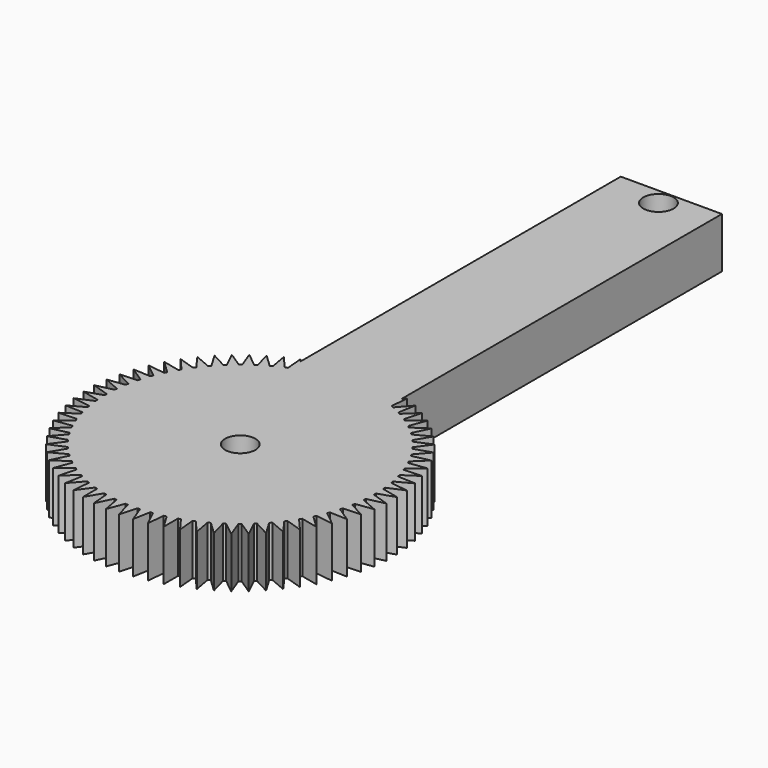
from build123d import *

# Parameters (mm, degrees)
F0_R     = 1.5
F1_DEPTH = 2.5
F3_DEPTH = 5


# Not quite as in the source:
# - a feature names something its author has since deleted; it is built from what else it names
# - the program builds the solid bodies; features that only make, move or delete a surface that nothing else refers to are left out


with BuildPart() as f1:
    # F0 (on Top) → F1 (new body, symmetric)
    with BuildSketch(Plane.XY):
        with BuildLine():
            Line((4.9747981783, 53.2882774979), (-5.0252018217, 53.2882774979))
            Line((-5.0252018217, 53.2882774979), (-5.0252018217, 14.1213197939))
            ThreePointArc((-5.0252018217, 14.1213197939), (-0.0267305738, 14.9880958204), (4.9747981783, 14.1391402048))
            Line((4.9747981783, 14.1391402048), (4.9747981783, 53.2882774979))
        make_face()
        with Locations((0, 51.666546613)):
            Circle(F0_R, mode=Mode.SUBTRACT)
        with BuildLine():
            ThreePointArc((4.9747981783, 14.1391402048), (-0.0267305738, 14.9880958204), (-5.0252018217, 14.1213197939))
            Line((-5.0252018217, 14.1213197939), (-5.0252018217, 13.7012252469))
            Line((-5.0252018217, 13.7012252469), (-5.2664479011, 14.0324002503))
            Line((-5.2664479011, 14.0324002503), (-5.1113713487, 12.2848828663))
            Line((-5.1113713487, 12.2848828663), (-5.35527293, 12.1933450718))
            Line((-5.35527293, 12.1933450718), (-6.5031013908, 13.5038291821))
            Line((-6.5031013908, 13.5038291821), (-6.1920028804, 11.7772477444))
            Line((-6.1920028804, 11.7772477444), (-6.4267172011, 11.6642152849))
            Line((-6.4267172011, 11.6642152849), (-7.6873957319, 12.8665332215))
            Line((-7.6873957319, 12.8665332215), (-7.2227800459, 11.1747891485))
            Line((-7.2227800459, 11.1747891485), (-7.4464173241, 11.0411720949))
            Line((-7.4464173241, 11.0411720949), (-8.8097956827, 12.1256435008))
            Line((-8.8097956827, 12.1256435008), (-8.1954036333, 10.482357721))
            Line((-8.1954036333, 10.482357721), (-8.4061632732, 10.3292318794))
            Line((-8.4061632732, 10.3292318794), (-9.8612643388, 11.2871252283))
            Line((-9.8612643388, 11.2871252283), (-9.1020426494, 9.7055285127))
            Line((-9.1020426494, 9.7055285127), (-9.2982277385, 9.5341267623))
            Line((-9.2982277385, 9.5341267623), (-10.8333358927, 10.3577296603))
            Line((-10.8333358927, 10.3577296603), (-9.9353973701, 8.8505560956))
            Line((-9.9353973701, 8.8505560956), (-10.1154283412, 8.6622584624))
            Line((-10.1154283412, 8.6622584624), (-11.7181837959, 9.3449397433))
            Line((-11.7181837959, 9.3449397433), (-10.6887581131, 7.9243242049))
            Line((-10.6887581131, 7.9243242049), (-10.8511854627, 7.7206467507))
            Line((-10.8511854627, 7.7206467507), (-12.5086837734, 8.2569098662))
            Line((-12.5086837734, 8.2569098662), (-11.3560592606, 6.934290315))
            Line((-11.3560592606, 6.934290315), (-11.4995752192, 6.7168729311))
            Line((-11.4995752192, 6.7168729311), (-13.1984711841, 7.1024002058))
            Line((-13.1984711841, 7.1024002058), (-11.9319280962, 5.8884255969))
            Line((-11.9319280962, 5.8884255969), (-12.0553771577, 5.6590188001))
            Line((-12.0553771577, 5.6590188001), (-13.7819922654, 5.8907061951))
            Line((-13.7819922654, 5.8907061951), (-12.4117280627, 4.7951507382))
            Line((-12.4117280627, 4.7951507382), (-12.5141162878, 4.5556015771))
            Line((-12.5141162878, 4.5556015771), (-14.2545488486, 4.6315836818))
            Line((-14.2545488486, 4.6315836818), (-12.7915960928, 3.6632681452))
            Line((-12.7915960928, 3.6632681452), (-12.8720991118, 3.4155053289))
            Line((-12.8720991118, 3.4155053289), (-14.6123361861, 3.3351703801))
            Line((-14.6123361861, 3.3351703801), (-13.0684737124, 2.5018910711))
            Line((-13.0684737124, 2.5018910711), (-13.1264433623, 2.2479094401))
            Line((-13.1264433623, 2.2479094401), (-14.8524735845, 2.0119042475))
            Line((-14.8524735845, 2.0119042475), (-13.2401316659, 1.3203702412))
            Line((-13.2401316659, 1.3203702412), (-13.2751012091, 1.0622147062))
            Line((-13.2751012091, 1.0622147062), (-14.9730275987, 0.6724394448))
            Line((-14.9730275987, 0.6724394448), (-13.3051878643, 0.1282185665))
            Line((-13.3051878643, 0.1282185665), (-13.3168757467, -0.132032356))
            Line((-13.3168757467, -0.132032356), (-14.9730275987, -0.6724394448))
            Line((-14.9730275987, -0.6724394448), (-13.2631185133, -1.0649654488))
            Line((-13.2631185133, -1.0649654488), (-13.2514306309, -1.3252163712))
            Line((-13.2514306309, -1.3252163712), (-14.8524735845, -2.0119042475))
            Line((-14.8524735845, -2.0119042475), (-13.1142623306, -2.2495749884))
            Line((-13.1142623306, -2.2495749884), (-13.0792927873, -2.5077305234))
            Line((-13.0792927873, -2.5077305234), (-14.6123361861, -3.3351703801))
            Line((-14.6123361861, -3.3351703801), (-12.8598178187, -3.4160722729))
            Line((-12.8598178187, -3.4160722729), (-12.8018481688, -3.670053904))
            Line((-12.8018481688, -3.670053904), (-14.2545488486, -4.6315836818))
            Line((-14.2545488486, -4.6315836818), (-12.5018336152, -4.5550653522))
            Line((-12.5018336152, -4.5550653522), (-12.4213305961, -4.8028281685))
            Line((-12.4213305961, -4.8028281685), (-13.7819922654, -5.8907061951))
            Line((-13.7819922654, -5.8907061951), (-12.0431919983, -5.6573837235))
            Line((-12.0431919983, -5.6573837235), (-11.9408037732, -5.8969328846))
            Line((-11.9408037732, -5.8969328846), (-13.1984711841, -7.1024002058))
            Line((-13.1984711841, -7.1024002058), (-11.4875856808, -6.7141521676))
            Line((-11.4875856808, -6.7141521676), (-11.3641366193, -6.9435589644))
            Line((-11.3641366193, -6.9435589644), (-12.5086837734, -8.2569098662))
            Line((-12.5086837734, -8.2569098662), (-10.839488078, -7.7168622063))
            Line((-10.839488078, -7.7168622063), (-10.6959721194, -7.9342795903))
            Line((-10.6959721194, -7.9342795903), (-11.7181837959, -9.3449397433))
            Line((-11.7181837959, -9.3449397433), (-10.1041172907, -8.657440608))
            Line((-10.1041172907, -8.657440608), (-9.9416899411, -8.8611180621))
            Line((-9.9416899411, -8.8611180621), (-10.8333358927, -10.3577296603))
            Line((-10.8333358927, -10.3577296603), (-9.287394092, -9.5283143883))
            Line((-9.287394092, -9.5283143883), (-9.107363121, -9.7166120216))
            Line((-9.107363121, -9.7166120216), (-9.8612643388, -11.2871252283))
            Line((-9.8612643388, -11.2871252283), (-8.3958942571, -10.3224717838))
            Line((-8.3958942571, -10.3224717838), (-8.1997091681, -10.4938735343))
            Line((-8.1997091681, -10.4938735343), (-8.8097956827, -12.1256435008))
            Line((-8.8097956827, -12.1256435008), (-7.4367956183, -11.033518706))
            Line((-7.4367956183, -11.033518706), (-7.2260359783, -11.1866445476))
            Line((-7.2260359783, -11.1866445476), (-7.6873957319, -12.8665332215))
            Line((-7.6873957319, -12.8665332215), (-6.4178202739, -11.6557302232))
            Line((-6.4178202739, -11.6557302232), (-6.1941829957, -11.7893472767))
            Line((-6.1941829957, -11.7893472767), (-6.5031013908, -13.5038291821))
            Line((-6.5031013908, -13.5038291821), (-5.3471724143, -12.184096654))
            Line((-5.3471724143, -12.184096654), (-5.1124580937, -12.2971291135))
            Line((-5.1124580937, -12.2971291135), (-5.2664479011, -14.0324002503))
            Line((-5.2664479011, -14.0324002503), (-4.2334722666, -12.6143639028))
            Line((-4.2334722666, -12.6143639028), (-3.9895706852, -12.7059016973))
            Line((-3.9895706852, -12.7059016973), (-3.9873920694, -14.4479906826))
            Line((-3.9873920694, -14.4479906826), (-3.0856866893, -12.9430677105))
            Line((-3.0856866893, -12.9430677105), (-2.8345615994, -13.0123738316))
            Line((-2.8345615994, -13.0123738316), (-2.6762321014, -14.7472543892))
            Line((-2.6762321014, -14.7472543892), (-1.9130569772, -13.1675615474))
            Line((-1.9130569772, -13.1675615474), (-1.6567302903, -13.214077983))
            Line((-1.6567302903, -13.214077983), (-1.3435246861, -14.9277818747))
            Line((-1.3435246861, -14.9277818747), (-0.7250244552, -13.2860379212))
            Line((-0.7250244552, -13.2860379212), (-0.465559963, -13.3093901482))
            Line((-0.465559963, -13.3093901482), (0, -14.9881196379))
            Line((0, -14.9881196379), (0.4688455374, -13.2975429296))
            Line((0.4688455374, -13.2975429296), (0.7293587793, -13.2975429296))
            Line((0.7293587793, -13.2975429296), (1.3435246861, -14.9277818747))
            Line((1.3435246861, -14.9277818747), (1.6589406614, -13.2019839413))
            Line((1.6589406614, -13.2019839413), (1.9184051536, -13.1786317143))
            Line((1.9184051536, -13.1786317143), (2.6762321014, -14.7472543892))
            Line((2.6762321014, -14.7472543892), (2.8356789707, -13.0001303408))
            Line((2.8356789707, -13.0001303408), (3.0920056577, -12.9536139053))
            Line((3.0920056577, -12.9536139053), (3.9873920694, -14.4479906826))
            Line((3.9873920694, -14.4479906826), (3.9895860602, -12.6936073349))
            Line((3.9895860602, -12.6936073349), (4.2407111502, -12.6243012138))
            Line((4.2407111502, -12.6243012138), (5.2664479011, -14.0324002503))
            Line((5.2664479011, -14.0324002503), (5.1113713487, -12.2848828663))
            Line((5.1113713487, -12.2848828663), (5.35527293, -12.1933450718))
            Line((5.35527293, -12.1933450718), (6.5031013908, -13.5038291821))
            Line((6.5031013908, -13.5038291821), (6.1920028804, -11.7772477444))
            Line((6.1920028804, -11.7772477444), (6.4267172011, -11.6642152849))
            Line((6.4267172011, -11.6642152849), (7.6873957319, -12.8665332215))
            Line((7.6873957319, -12.8665332215), (7.2227800459, -11.1747891485))
            Line((7.2227800459, -11.1747891485), (7.4464173241, -11.0411720949))
            Line((7.4464173241, -11.0411720949), (8.8097956827, -12.1256435008))
            Line((8.8097956827, -12.1256435008), (8.1954036333, -10.482357721))
            Line((8.1954036333, -10.482357721), (8.4061632732, -10.3292318794))
            Line((8.4061632732, -10.3292318794), (9.8612643388, -11.2871252283))
            Line((9.8612643388, -11.2871252283), (9.1020426494, -9.7055285127))
            Line((9.1020426494, -9.7055285127), (9.2982277385, -9.5341267623))
            Line((9.2982277385, -9.5341267623), (10.8333358927, -10.3577296603))
            Line((10.8333358927, -10.3577296603), (9.9353973701, -8.8505560956))
            Line((9.9353973701, -8.8505560956), (10.1154283412, -8.6622584624))
            Line((10.1154283412, -8.6622584624), (11.7181837959, -9.3449397433))
            Line((11.7181837959, -9.3449397433), (10.6887581131, -7.9243242049))
            Line((10.6887581131, -7.9243242049), (10.8511854627, -7.7206467507))
            Line((10.8511854627, -7.7206467507), (12.5086837734, -8.2569098662))
            Line((12.5086837734, -8.2569098662), (11.3560592606, -6.934290315))
            Line((11.3560592606, -6.934290315), (11.4995752192, -6.7168729311))
            Line((11.4995752192, -6.7168729311), (13.1984711841, -7.1024002058))
            Line((13.1984711841, -7.1024002058), (11.9319280962, -5.8884255969))
            Line((11.9319280962, -5.8884255969), (12.0553771577, -5.6590188001))
            Line((12.0553771577, -5.6590188001), (13.7819922654, -5.8907061951))
            Line((13.7819922654, -5.8907061951), (12.4117280627, -4.7951507382))
            Line((12.4117280627, -4.7951507382), (12.5141162878, -4.5556015771))
            Line((12.5141162878, -4.5556015771), (14.2545488486, -4.6315836818))
            Line((14.2545488486, -4.6315836818), (12.7915960928, -3.6632681452))
            Line((12.7915960928, -3.6632681452), (12.8720991118, -3.4155053289))
            Line((12.8720991118, -3.4155053289), (14.6123361861, -3.3351703801))
            Line((14.6123361861, -3.3351703801), (13.0684737124, -2.5018910711))
            Line((13.0684737124, -2.5018910711), (13.1264433623, -2.2479094401))
            Line((13.1264433623, -2.2479094401), (14.8524735845, -2.0119042475))
            Line((14.8524735845, -2.0119042475), (13.2401316659, -1.3203702412))
            Line((13.2401316659, -1.3203702412), (13.2751012091, -1.0622147062))
            Line((13.2751012091, -1.0622147062), (14.9730275987, -0.6724394448))
            Line((14.9730275987, -0.6724394448), (13.3051878643, -0.1282185665))
            Line((13.3051878643, -0.1282185665), (13.3168757467, 0.132032356))
            Line((13.3168757467, 0.132032356), (14.9730275987, 0.6724394448))
            Line((14.9730275987, 0.6724394448), (13.2631185133, 1.0649654488))
            Line((13.2631185133, 1.0649654488), (13.2514306309, 1.3252163712))
            Line((13.2514306309, 1.3252163712), (14.8524735845, 2.0119042475))
            Line((14.8524735845, 2.0119042475), (13.1142623306, 2.2495749884))
            Line((13.1142623306, 2.2495749884), (13.0792927873, 2.5077305234))
            Line((13.0792927873, 2.5077305234), (14.6123361861, 3.3351703801))
            Line((14.6123361861, 3.3351703801), (12.8598178187, 3.4160722729))
            Line((12.8598178187, 3.4160722729), (12.8018481688, 3.670053904))
            Line((12.8018481688, 3.670053904), (14.2545488486, 4.6315836818))
            Line((14.2545488486, 4.6315836818), (12.5018336152, 4.5550653522))
            Line((12.5018336152, 4.5550653522), (12.4213305961, 4.8028281685))
            Line((12.4213305961, 4.8028281685), (13.7819922654, 5.8907061951))
            Line((13.7819922654, 5.8907061951), (12.0431919983, 5.6573837235))
            Line((12.0431919983, 5.6573837235), (11.9408037732, 5.8969328846))
            Line((11.9408037732, 5.8969328846), (13.1984711841, 7.1024002058))
            Line((13.1984711841, 7.1024002058), (11.4875856808, 6.7141521676))
            Line((11.4875856808, 6.7141521676), (11.3641366193, 6.9435589644))
            Line((11.3641366193, 6.9435589644), (12.5086837734, 8.2569098662))
            Line((12.5086837734, 8.2569098662), (10.839488078, 7.7168622063))
            Line((10.839488078, 7.7168622063), (10.6959721194, 7.9342795903))
            Line((10.6959721194, 7.9342795903), (11.7181837959, 9.3449397433))
            Line((11.7181837959, 9.3449397433), (10.1041172907, 8.657440608))
            Line((10.1041172907, 8.657440608), (9.9416899411, 8.8611180621))
            Line((9.9416899411, 8.8611180621), (10.8333358927, 10.3577296603))
            Line((10.8333358927, 10.3577296603), (9.287394092, 9.5283143883))
            Line((9.287394092, 9.5283143883), (9.107363121, 9.7166120216))
            Line((9.107363121, 9.7166120216), (9.8612643388, 11.2871252283))
            Line((9.8612643388, 11.2871252283), (8.3958942571, 10.3224717838))
            Line((8.3958942571, 10.3224717838), (8.1997091681, 10.4938735343))
            Line((8.1997091681, 10.4938735343), (8.8097956827, 12.1256435008))
            Line((8.8097956827, 12.1256435008), (7.4367956183, 11.033518706))
            Line((7.4367956183, 11.033518706), (7.2260359783, 11.1866445476))
            Line((7.2260359783, 11.1866445476), (7.6873957319, 12.8665332215))
            Line((7.6873957319, 12.8665332215), (6.4178202739, 11.6557302232))
            Line((6.4178202739, 11.6557302232), (6.1941829957, 11.7893472767))
            Line((6.1941829957, 11.7893472767), (6.5031013908, 13.5038291821))
            Line((6.5031013908, 13.5038291821), (5.3471724143, 12.184096654))
            Line((5.3471724143, 12.184096654), (5.1124580937, 12.2971291135))
            Line((5.1124580937, 12.2971291135), (5.2664479011, 14.0324002503))
            Line((5.2664479011, 14.0324002503), (4.9747981783, 13.6320327162))
            Line((4.9747981783, 13.6320327162), (4.9747981783, 14.1391402048))
        make_face()
        Circle(F0_R, mode=Mode.SUBTRACT)
    extrude(amount=F1_DEPTH, both=True)

    # F0 (on Top) → F3 (join)
    with BuildSketch(Plane.XY):
        with Locations((0, 51.666546613)):
            Circle(F0_R)
        Circle(F0_R)
    extrude(amount=-F3_DEPTH)


solid = f1.part
